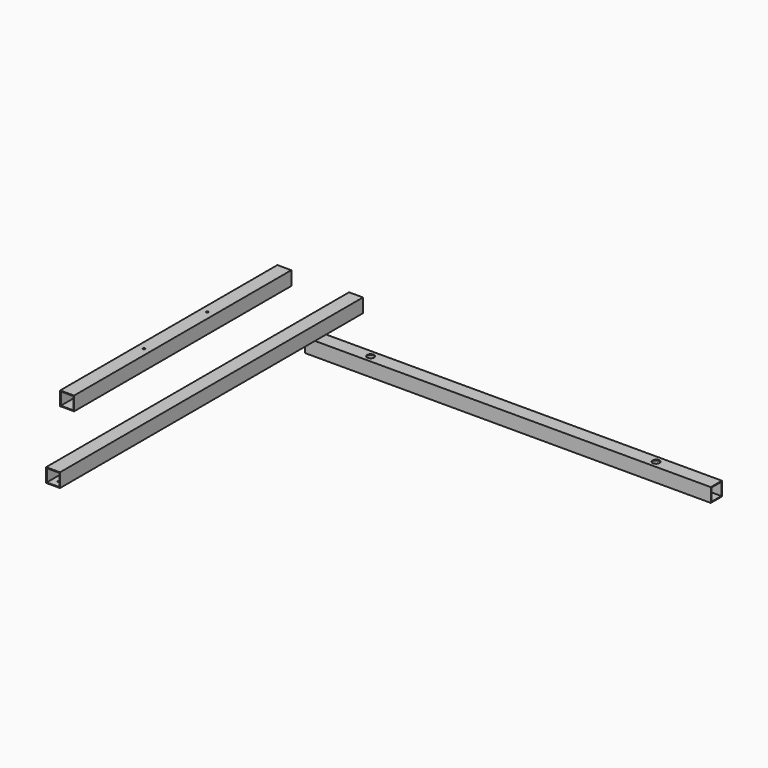
from build123d import *

# Parameters (mm, degrees)
F0_W      = 20
F0_H      = 20
F0_W_2    = 18
F0_H_2    = 18
F1_DEPTH  = 390
F2_R      = 1.55
F3_DEPTH  = 20
F4_W      = 20
F4_H      = 20
F4_W_2    = 18
F4_H_2    = 18
F5_DEPTH  = 583
F6_R      = 5.1
F7_DEPTH  = 20.001
F8_W      = 20
F8_H      = 20
F8_W_2    = 18
F8_H_2    = 18
F9_DEPTH  = 544
F10_R     = 1.6
F11_DEPTH = 1


# Not quite as in the source:
# - a feature names something its author has since deleted; it is built from what else it names


with BuildPart() as f1:
    # F0 (on Front) → F1 (new body)
    with BuildSketch(Plane.XZ):
        with Locations((-64.8252740502, 40.6123196004)):
            Rectangle(F0_W, F0_H)
        with Locations((-64.8252740502, 40.6123196004)):
            Rectangle(F0_W_2, F0_H_2, mode=Mode.SUBTRACT)
    extrude(amount=F1_DEPTH)

    # F2 (on face) → F3 (cut, through all)
    with BuildSketch(Plane.XY.offset(50.6123196004)):
        with Locations((-64.8252740502, -138)):
            Circle(F2_R)
        with Locations((-64.8252740502, -252)):
            Circle(F2_R)
    extrude(amount=-F3_DEPTH, mode=Mode.SUBTRACT)


with BuildPart() as f5:
    # F4 (on Right) → F5 (new body)
    with BuildSketch(Plane.YZ):
        with Locations((-34.0558066964, -8.3925398067)):
            Rectangle(F4_W, F4_H)
        with Locations((-34.0558066964, -8.3925398067)):
            Rectangle(F4_W_2, F4_H_2, mode=Mode.SUBTRACT)
    extrude(amount=F5_DEPTH)

    # F6 (on face) → F7 (cut, through all)
    with BuildSketch(Plane.XY.offset(1.6074601933)):
        with Locations((86.5, -34.0558066964)):
            Circle(F6_R)
        with Locations((496.5, -34.0558066964)):
            Circle(F6_R)
    extrude(amount=-F7_DEPTH, mode=Mode.SUBTRACT)


with BuildPart() as f9:
    # F8 (on Front) → F9 (new body)
    with BuildSketch(Plane.XZ):
        with Locations((38.1599590182, 39.6779589355)):
            Rectangle(F8_W, F8_H)
        with Locations((38.1599590182, 39.6779589355)):
            Rectangle(F8_W_2, F8_H_2, mode=Mode.SUBTRACT)
    extrude(amount=F9_DEPTH)

    # F10 (on face) → F11 (cut, through all)
    with BuildSketch(Plane(origin=(0, 0, 29.6779589355), x_dir=(1, 0, 0), z_dir=(0, 0, -1))):
        with Locations((38.1599590182, 10)):
            Circle(F10_R)
        with Locations((38.1599590182, 50)):
            Circle(F10_R)
        with Locations((38.1599590182, 494)):
            Circle(F10_R)
        with Locations((38.1599590182, 534)):
            Circle(F10_R)
    extrude(amount=-F11_DEPTH, mode=Mode.SUBTRACT)


solid = Compound([f1.part, f5.part, f9.part])
